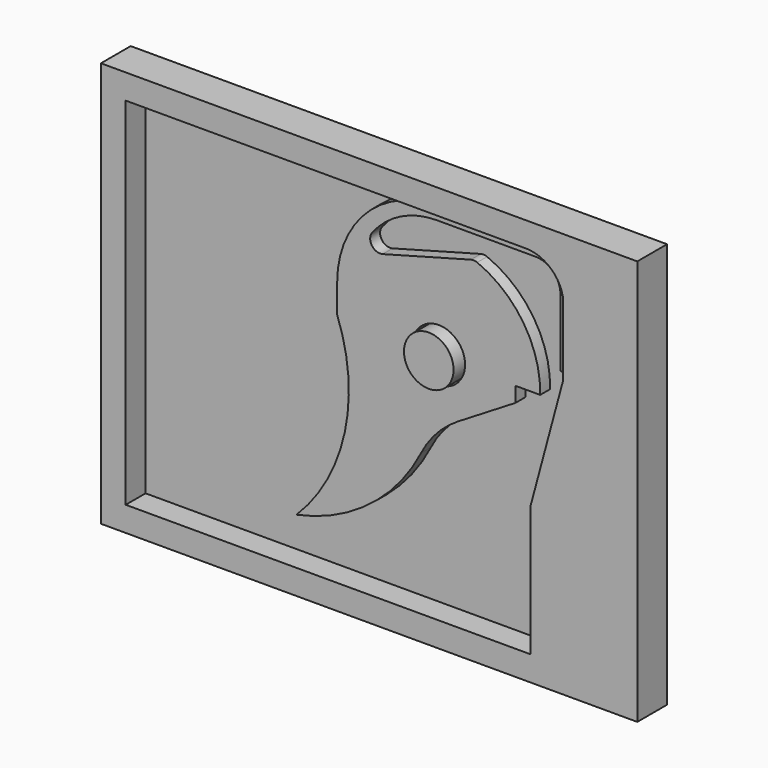
from build123d import *

# Parameters (mm, degrees)
F0_R     = 3.3782
F1_DEPTH = 1.5875
F2_R     = 1.27
F0_W     = 68.6608534306
F0_H     = 51.8983377281
F0_R_2   = 3.175
F3_DEPTH = 1.5875
F4_DEPTH = 3.175


with BuildPart() as f1:
    # F0 (on Front) → F1 (new body)
    with BuildSketch(Plane.XZ):
        with BuildLine():
            Line((37.0810907311, 22.1493569333), (44.45, 26.6400993653))
            Line((44.45, 26.6400993653), (44.45, 28.575))
            Line((44.45, 28.575), (47.625, 28.575))
            ThreePointArc((47.625, 28.575), (45.3798217244, 36.1628892804), (39.1499755584, 41.0420189125))
            Line((39.1499755584, 41.0420189125), (24.5960312701, 37.1132397757))
            ThreePointArc((24.5960312701, 37.1132397757), (28.4208043201, 42.0794558253), (34.4001515145, 43.9608377281))
            Line((34.4001515145, 43.9608377281), (47.0392336093, 43.9608377281))
            Line((47.0392336093, 43.9608377281), (47.0392336093, 45.5483377281))
            Line((47.0392336093, 45.5483377281), (34.3392336093, 45.5483377281))
            ThreePointArc((34.3392336093, 45.5483377281), (25.3589774882, 41.8285938491), (21.6392336093, 32.8483377281))
            Line((21.6392336093, 32.8483377281), (21.6392336093, 29.1382938078))
            ThreePointArc((21.6392336093, 29.1382938078), (22.6164587492, 16.2619847329), (16.4273683424, 4.9284299373))
            ThreePointArc((16.4273683424, 4.9284299373), (25.7864104877, 9.1668684971), (32.3673924103, 17.0565268063))
            ThreePointArc((32.3673924103, 17.0565268063), (34.369647916, 19.9311380738), (37.0810907311, 22.1493569333))
        make_face()
        with Locations((34.6321168046, 28.8566469039)):
            Circle(F0_R, mode=Mode.SUBTRACT)
        with BuildLine():
            Line((50.2142336093, 32.1144140998), (51.8017336093, 32.1144140998))
            Line((51.8017336093, 32.1144140998), (51.8017336093, 41.6394140998))
            ThreePointArc((51.8017336093, 41.6394140998), (50.1198622051, 44.4459750797), (47.0392336093, 45.5483377281))
            Line((47.0392336093, 45.5483377281), (47.0392336093, 43.9608377281))
            ThreePointArc((47.0392336093, 43.9608377281), (49.2842976395, 43.0309017583), (50.2142336093, 40.7858377281))
            Line((50.2142336093, 40.7858377281), (50.2142336093, 32.1144140998))
        make_face()
    extrude(amount=F1_DEPTH)

    # F2
    f2_edges = [f1.edges().sort_by_distance(p)[0] for p in [
        (24.596031, -0.79375, 37.11324),
        (39.149976, -0.79375, 41.042019),
    ]]
    fillet(f2_edges, radius=F2_R)


with BuildPart() as f3:
    # F0 (on Front) → F3 (new body)
    with BuildSketch(Plane.XZ):
        with Locations((26.9963068939, 22.774168864)):
            Rectangle(F0_W, F0_H)
        Polygon((47.625, 0), (0, 0), (-4.1591198214, 0), (-4.1591198214, 45.5483377281), (34.3392336093, 45.5483377281), (47.0392336093, 45.5483377281), (58.1517336093, 45.5483377281), (58.1517336093, 0), align=None, mode=Mode.SUBTRACT)
        with BuildLine():
            Line((-4.1591198214, 0), (0, 0))
            Line((0, 0), (47.625, 0))
            Line((47.625, 0), (47.625, 16.5848955512))
            Line((47.625, 16.5848955512), (44.45, 26.6400993653))
            Line((44.45, 26.6400993653), (37.0810907311, 22.1493569333))
            ThreePointArc((37.0810907311, 22.1493569333), (34.369647916, 19.9311380738), (32.3673924103, 17.0565268063))
            ThreePointArc((32.3673924103, 17.0565268063), (25.7864104877, 9.1668684971), (16.4273683424, 4.9284299373))
            ThreePointArc((16.4273683424, 4.9284299373), (22.6164587492, 16.2619847329), (21.6392336093, 29.1382938078))
            Line((21.6392336093, 29.1382938078), (21.6392336093, 32.8483377281))
            ThreePointArc((21.6392336093, 32.8483377281), (25.3589774882, 41.8285938491), (34.3392336093, 45.5483377281))
            Line((34.3392336093, 45.5483377281), (-4.1591198214, 45.5483377281))
            Line((-4.1591198214, 45.5483377281), (-4.1591198214, 0))
        make_face()
        with BuildLine():
            Line((37.0810907311, 22.1493569333), (44.45, 26.6400993653))
            Line((44.45, 26.6400993653), (44.45, 28.575))
            Line((44.45, 28.575), (47.625, 28.575))
            ThreePointArc((47.625, 28.575), (45.3798217244, 36.1628892804), (39.1499755584, 41.0420189125))
            Line((39.1499755584, 41.0420189125), (24.5960312701, 37.1132397757))
            ThreePointArc((24.5960312701, 37.1132397757), (28.4208043201, 42.0794558253), (34.4001515145, 43.9608377281))
            Line((34.4001515145, 43.9608377281), (47.0392336093, 43.9608377281))
            Line((47.0392336093, 43.9608377281), (47.0392336093, 45.5483377281))
            Line((47.0392336093, 45.5483377281), (34.3392336093, 45.5483377281))
            ThreePointArc((34.3392336093, 45.5483377281), (25.3589774882, 41.8285938491), (21.6392336093, 32.8483377281))
            Line((21.6392336093, 32.8483377281), (21.6392336093, 29.1382938078))
            ThreePointArc((21.6392336093, 29.1382938078), (22.6164587492, 16.2619847329), (16.4273683424, 4.9284299373))
            ThreePointArc((16.4273683424, 4.9284299373), (25.7864104877, 9.1668684971), (32.3673924103, 17.0565268063))
            ThreePointArc((32.3673924103, 17.0565268063), (34.369647916, 19.9311380738), (37.0810907311, 22.1493569333))
        make_face()
        with Locations((34.6321168046, 28.8566469039)):
            Circle(F0_R, mode=Mode.SUBTRACT)
        with BuildLine():
            Line((47.625, 16.5848955512), (47.625, 0))
            Line((47.625, 0), (58.1517336093, 0))
            Line((58.1517336093, 0), (58.1517336093, 45.5483377281))
            Line((58.1517336093, 45.5483377281), (47.0392336093, 45.5483377281))
            ThreePointArc((47.0392336093, 45.5483377281), (50.1198622051, 44.4459750797), (51.8017336093, 41.6394140998))
            Line((51.8017336093, 41.6394140998), (51.8017336093, 32.1144140998))
            Line((51.8017336093, 32.1144140998), (47.625, 16.5848955512))
        make_face()
        with BuildLine():
            Line((44.45, 26.6400993653), (47.625, 16.5848955512))
            Line((47.625, 16.5848955512), (51.8017336093, 32.1144140998))
            Line((51.8017336093, 32.1144140998), (50.2142336093, 32.1144140998))
            Line((50.2142336093, 32.1144140998), (50.2142336093, 40.7858377281))
            ThreePointArc((50.2142336093, 40.7858377281), (49.2842976395, 43.0309017583), (47.0392336093, 43.9608377281))
            Line((47.0392336093, 43.9608377281), (34.4001515145, 43.9608377281))
            ThreePointArc((34.4001515145, 43.9608377281), (28.4208043201, 42.0794558253), (24.5960312701, 37.1132397757))
            Line((24.5960312701, 37.1132397757), (39.1499755584, 41.0420189125))
            ThreePointArc((39.1499755584, 41.0420189125), (45.3798217244, 36.1628892804), (47.625, 28.575))
            Line((47.625, 28.575), (44.45, 28.575))
            Line((44.45, 28.575), (44.45, 26.6400993653))
        make_face()
        with Locations((34.6321168046, 28.8566469039)):
            Circle(F0_R)
        with Locations((34.6321168046, 28.8566469039)):
            Circle(F0_R_2, mode=Mode.SUBTRACT)
        with Locations((34.6321168046, 28.8566469039)):
            Circle(F0_R_2)
        with BuildLine():
            Line((50.2142336093, 32.1144140998), (51.8017336093, 32.1144140998))
            Line((51.8017336093, 32.1144140998), (51.8017336093, 41.6394140998))
            ThreePointArc((51.8017336093, 41.6394140998), (50.1198622051, 44.4459750797), (47.0392336093, 45.5483377281))
            Line((47.0392336093, 45.5483377281), (47.0392336093, 43.9608377281))
            ThreePointArc((47.0392336093, 43.9608377281), (49.2842976395, 43.0309017583), (50.2142336093, 40.7858377281))
            Line((50.2142336093, 40.7858377281), (50.2142336093, 32.1144140998))
        make_face()
    extrude(amount=-F3_DEPTH)

    # F0 (on Front) → F4 (join)
    with BuildSketch(Plane.XZ):
        with Locations((26.9963068939, 22.774168864)):
            Rectangle(F0_W, F0_H)
        Polygon((47.625, 0), (0, 0), (-4.1591198214, 0), (-4.1591198214, 45.5483377281), (34.3392336093, 45.5483377281), (47.0392336093, 45.5483377281), (58.1517336093, 45.5483377281), (58.1517336093, 0), align=None, mode=Mode.SUBTRACT)
        with Locations((34.6321168046, 28.8566469039)):
            Circle(F0_R_2)
        with BuildLine():
            Line((47.625, 16.5848955512), (47.625, 0))
            Line((47.625, 0), (58.1517336093, 0))
            Line((58.1517336093, 0), (58.1517336093, 45.5483377281))
            Line((58.1517336093, 45.5483377281), (47.0392336093, 45.5483377281))
            ThreePointArc((47.0392336093, 45.5483377281), (50.1198622051, 44.4459750797), (51.8017336093, 41.6394140998))
            Line((51.8017336093, 41.6394140998), (51.8017336093, 32.1144140998))
            Line((51.8017336093, 32.1144140998), (47.625, 16.5848955512))
        make_face()
    extrude(amount=F4_DEPTH)


solid = Compound([f1.part, f3.part])
